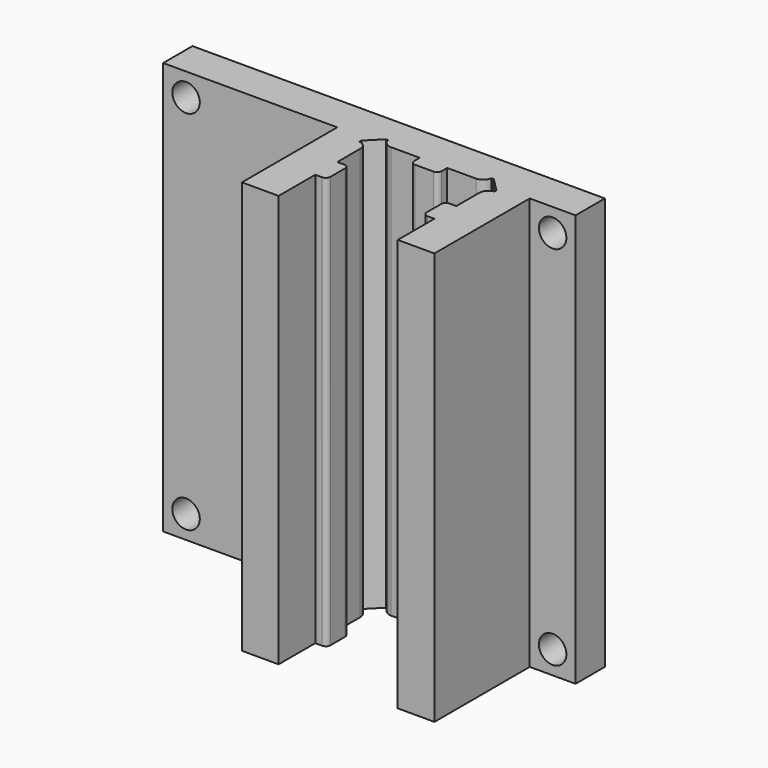
from build123d import *

# Parameters (mm, degrees)
F1_DEPTH     = 90
F2_R         = 3
F3_DEPTH     = 25
F4_W         = 3.5
F4_H         = 3.5
F5_DEPTH     = 300
F6_SIZE      = 3
F7_SIZE      = 3
F8_R         = 1
F9_T1_DEPTH  = 99.9215674165
F10_T1_DEPTH = 99.9215674165


# Not quite as in the source:
# - a fillet or chamfer that OpenCascade refuses, or shapes differently, is made with other operations: its cross-section is extruded or revolved along the edge and cut away or added


with BuildPart() as f1:
    # F0 (on Top) → F1 (new body)
    with BuildSketch(Plane.XY):
        Polygon((0, 26), (0, 0), (8, 0), (8, 10), (10.5, 10), (10.5, 16), (8, 16), (8, 26), (18, 26), (18, 23.5), (24, 23.5), (24, 26), (34, 26), (34, 16), (31.5, 16), (31.5, 10), (34, 10), (34, 0), (42, 0), (42, 26), (52, 26), (52, 34), (-38, 34), (-38, 26), align=None)
    extrude(amount=F1_DEPTH)

    # F2 (on face) → F3 (cut)
    with BuildSketch(Plane(origin=(0, 34, 0), x_dir=(-1, 0, 0), z_dir=(0, 1, 0))):
        with Locations((33, 85)):
            Circle(F2_R)
        with Locations((33, 5)):
            Circle(F2_R)
        with Locations((-47, 5)):
            Circle(F2_R)
        with Locations((-47, 85)):
            Circle(F2_R)
    extrude(amount=-F3_DEPTH, mode=Mode.SUBTRACT)

    # F4 (on face) → F5 (cut)
    with BuildSketch(Plane.XY.offset(90)):
        with Locations((8, 26)):
            Rectangle(F4_W, F4_H)
        with Locations((34, 26)):
            Rectangle(F4_W, F4_H)
    extrude(amount=-F5_DEPTH, mode=Mode.SUBTRACT)

    # F6
    f6_edges = [f1.edges().sort_by_distance(p)[0] for p in [
        (6.25, 27.75, 45),
    ]]
    chamfer(f6_edges, length=F6_SIZE)

    # F7
    f7_edges = [f1.edges().sort_by_distance(p)[0] for p in [
        (35.75, 27.75, 45),
    ]]
    chamfer(f7_edges, length=F7_SIZE)

    # F8
    f8_edges = [f1.edges().sort_by_distance(p)[0] for p in [
        (10.5, 10, 45),
        (10.5, 16, 45),
        (18, 23.5, 45),
        (24, 23.5, 45),
        (31.5, 10, 45),
        (31.5, 16, 45),
    ]]
    fillet(f8_edges, radius=F8_R)

    # F9: fillet of radius 2 on 2 edges, made by hand

    # F9_s2 → F9_t1 (cut)
    with BuildSketch(Plane.XY.offset(-4.9607837082)):
        with BuildLine():
            ThreePointArc((35.75, 24.25), (34.5, 23.5885621722), (34, 22.2656865167))
            Line((34, 22.2656865167), (34, 24.25))
            Line((34, 24.25), (35.75, 24.25))
        make_face()
        with BuildLine():
            ThreePointArc((30.2656865167, 26), (31.5885621722, 26.5), (32.25, 27.75))
            Line((32.25, 27.75), (32.25, 26))
            Line((32.25, 26), (30.2656865167, 26))
        make_face()
    extrude(amount=F9_T1_DEPTH, mode=Mode.SUBTRACT)

    # F10: fillet of radius 2 on 2 edges, made by hand

    # F10_s2 → F10_t1 (cut)
    with BuildSketch(Plane.XY.offset(-4.9607837082)):
        with BuildLine():
            ThreePointArc((11.7343134833, 26), (10.4114378278, 26.5), (9.75, 27.75))
            Line((9.75, 27.75), (9.75, 26))
            Line((9.75, 26), (11.7343134833, 26))
        make_face()
        with BuildLine():
            ThreePointArc((6.25, 24.25), (7.5, 23.5885621722), (8, 22.2656865167))
            Line((8, 22.2656865167), (8, 24.25))
            Line((8, 24.25), (6.25, 24.25))
        make_face()
    extrude(amount=F10_T1_DEPTH, mode=Mode.SUBTRACT)


solid = f1.part
